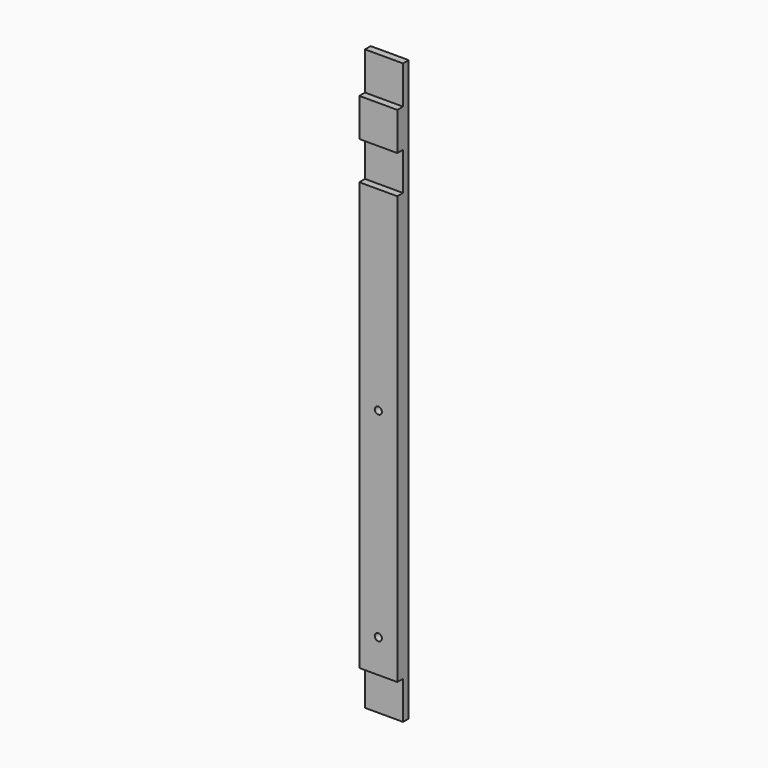
from build123d import *

# Parameters (mm, degrees)
F0_W     = 50.8
F0_H     = 19.05
F1_DEPTH = 774.7
F2_W     = 122.43557321
F2_H     = 50.8
F2_W_2   = 343.1604206562
F2_W_3   = 253.376558423
F3_DEPTH = 25.4
F4_R     = 0.79375
F5_DEPTH = 25.4
F6_R     = 4.7625
F7_DEPTH = 25.4


# Not quite as in the source:
# - a feature names something its author has since deleted; it is built from what else it names


with BuildPart() as f1:
    # F0 (on Top) → F1 (new body)
    with BuildSketch(Plane.XY):
        Rectangle(F0_W, F0_H)
    extrude(amount=F1_DEPTH)

    # F2 (on Front) → F3 (cut)
    with BuildSketch(Plane.XZ):
        with Locations((22.4465244144, 25.4)):
            Rectangle(F2_W, F2_H)
        with Locations((-38.7818217278, 749.3)):
            Rectangle(F2_W_2, F2_H)
        with Locations((-33.7835475802, 647.7)):
            Rectangle(F2_W_3, F2_H)
    extrude(amount=F3_DEPTH, mode=Mode.SUBTRACT)

    # F4 (on Front) → F5 (cut)
    with BuildSketch(Plane.XZ):
        with Locations((9.525, 101.6)):
            Circle(F4_R)
        with Locations((9.525, 155.575)):
            Circle(F4_R)
        with Locations((9.525, 619.125)):
            Circle(F4_R)
        with Locations((9.525, 673.1)):
            Circle(F4_R)
        with Locations((-9.525, 619.125)):
            Circle(F4_R)
        with Locations((-9.525, 673.1)):
            Circle(F4_R)
        with Locations((-9.525, 101.6)):
            Circle(F4_R)
        with Locations((-9.525, 155.575)):
            Circle(F4_R)
    extrude(amount=-F5_DEPTH, mode=Mode.SUBTRACT)

    # F6 (on Front) → F7 (cut)
    with BuildSketch(Plane.XZ):
        with Locations((0, 95.25)):
            Circle(F6_R)
        with Locations((0, 361.95)):
            Circle(F6_R)
    extrude(amount=F7_DEPTH, mode=Mode.SUBTRACT)


solid = f1.part
